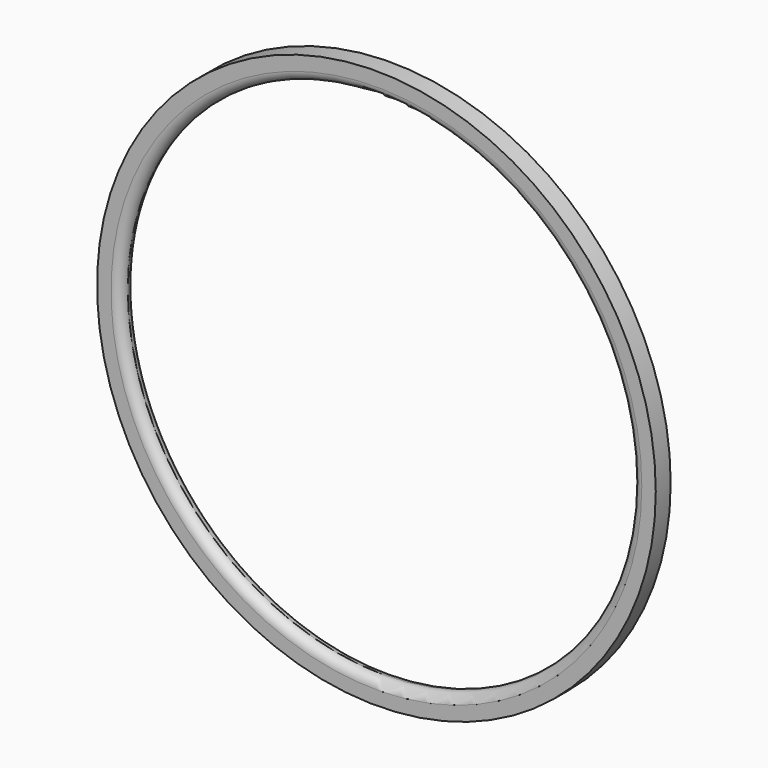
from build123d import *

# Parameters (mm, degrees)
F0_R     = 76.2
F0_R_2   = 69.85
F1_DEPTH = 5.08
F2_R     = 2.53999


# Not quite as in the source:
# - a fillet or chamfer is up to 0.001 mm smaller than in the source, because OpenCascade refuses the exact size


with BuildPart() as f1:
    # F0 (on Front) → F1 (new body)
    with BuildSketch(Plane.XZ):
        Circle(F0_R)
        Circle(F0_R_2, mode=Mode.SUBTRACT)
    extrude(amount=F1_DEPTH)

    # F2 (radius 2.54 in the source; OpenCascade refuses exactly that, so slightly less here)
    f2_edges = [f1.edges().sort_by_distance(p)[0] for p in [
        (-69.85, -5.08, 0),
        (-69.85, 0, 0),
    ]]
    fillet(f2_edges, radius=F2_R)


solid = f1.part
